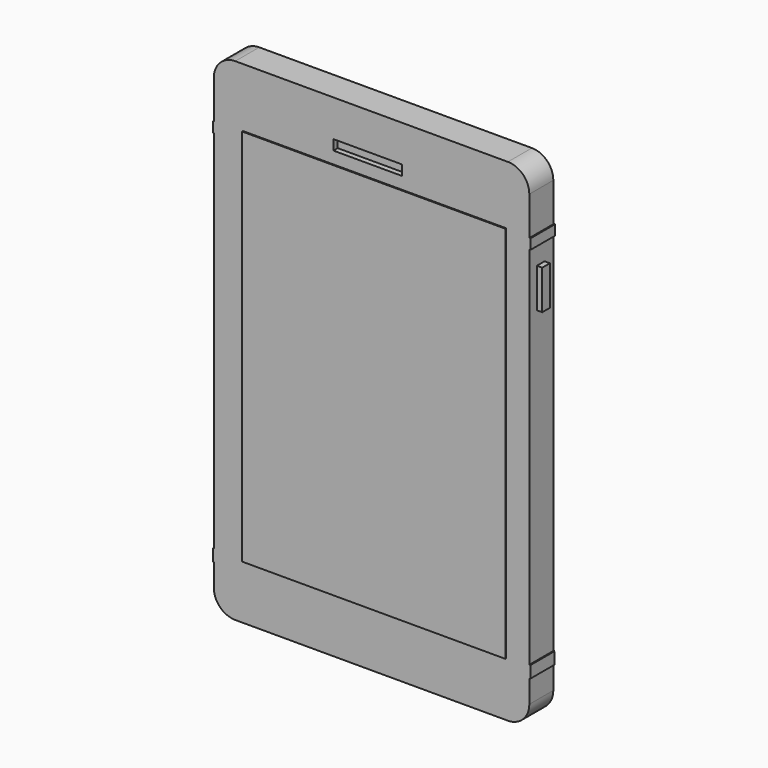
from build123d import *

# Parameters (mm, degrees)
F0_W      = 74.7929699719
F0_H      = 116.6311837733
F1_DEPTH  = 7.112
F2_W      = 2.2798741702
F2_H      = 9.3019269407
F3_DEPTH  = 1.27
F4_W      = 1.6649477184
F4_H      = 7.7697578818
F5_DEPTH  = 1.27
F4_H_2    = 7.214775309
F6_DEPTH  = 1.27
F4_W_2    = 1.2949595693
F4_H_3    = 4.4398605824
F7_DEPTH  = 0.508
F10_W     = 16.2794925272
F10_H     = 2.4049207568
F11_DEPTH = 1.27
F14_R     = 5.08
F15_R     = 5.08
F16_W     = 62.410261482
F16_H     = 89.7654034197
F17_DEPTH = 0.254
F21_R     = 5.3775746227
F22_DEPTH = 0.254
F25_W     = 74.7929699719
F25_H     = 2.4049244821
F26_DEPTH = 0.254
F29_DEPTH = 0.254
F30_DEPTH = 0.254
F31_W     = 74.7929699719
F31_H     = 2.9377117753
F34_DEPTH = 0.254
F32_W     = 7.112
F32_H     = 2.813577652
F35_DEPTH = 0.254
F33_W     = 7.112
F33_H     = 2.8514191508
F36_DEPTH = 0.254
F8_R      = 0.7916480681
F39_DEPTH = 1.27
F9_R      = 0.7862255443
F9_R_2    = 0.7916480681
F9_R_3    = 0.7862255169
F9_R_4    = 0.7902964021
F40_DEPTH = 1.27
F41_W     = 7.3253975715
F41_H     = 1.6351337545
F42_DEPTH = 1.27


# Not quite as in the source:
# - the program builds the solid bodies; features that only make, move or delete a surface that nothing else refers to are left out


with BuildPart() as f1:
    # F0 (on Front) → F1 (new body)
    with BuildSketch(Plane.XZ):
        with Locations((0.7164049894, -7.1640815586)):
            Rectangle(F0_W, F0_H)
    extrude(amount=F1_DEPTH)

    # F2 (on face) → F3 (join)
    with BuildSketch(Plane.YZ.offset(38.1128899753)):
        with Locations((-3.7364399759, 25.567272678)):
            Rectangle(F2_W, F2_H)
    extrude(amount=F3_DEPTH)

    # F4 (on face) → F5 (join)
    with BuildSketch(Plane(origin=(-36.6800799966, 0, 0), x_dir=(0, -1, 0), z_dir=(-1, 0, 0))):
        with Locations((2.8674099594, 15.4470177367)):
            Rectangle(F4_W, F4_H)
    extrude(amount=F5_DEPTH)

    # F4 (on face) → F6 (join)
    with BuildSketch(Plane(origin=(-36.6800799966, 0, 0), x_dir=(0, -1, 0), z_dir=(-1, 0, 0))):
        with Locations((2.8674099594, 27.5641391054)):
            Rectangle(F4_W, F4_H_2)
    extrude(amount=F6_DEPTH)

    # F4 (on face) → F7 (join)
    with BuildSketch(Plane(origin=(-36.6800799966, 0, 0), x_dir=(0, -1, 0), z_dir=(-1, 0, 0))):
        with Locations((3.052404034, 38.941282779)):
            Rectangle(F4_W_2, F4_H_3)
    extrude(amount=F7_DEPTH)

    # F10 (on face) → F11 (cut)
    with BuildSketch(Plane.XZ.offset(7.112)):
        with Locations((-0.1849941909, 41.2537120283)):
            Rectangle(F10_W, F10_H)
    extrude(amount=-F11_DEPTH, mode=Mode.SUBTRACT)

    # F14
    f14_edges = [f1.edges().sort_by_distance(p)[0] for p in [
        (38.11289, -3.556, 51.15151),
    ]]
    fillet(f14_edges, radius=F14_R)

    # F15
    f15_edges = [f1.edges().sort_by_distance(p)[0] for p in [
        (-36.68008, -3.556, 51.15151),
        (-36.68008, -3.556, -65.479673),
        (38.11289, -3.556, -65.479673),
    ]]
    fillet(f15_edges, radius=F15_R)

    # F16 (on face) → F17 (join)
    with BuildSketch(Plane.XZ.offset(7.112)):
        with Locations((1.43471919, -7.7157635242)):
            Rectangle(F16_W, F16_H)
    extrude(amount=F17_DEPTH)

    # F21 (on Front) → F22 (join)
    with BuildSketch(Plane.XZ):
        with Locations((30.1540587097, 43.5661412776)):
            Circle(F21_R)
    extrude(amount=-F22_DEPTH)

    # F25 (on face) → F26 (join)
    with BuildSketch(Plane(origin=(0, 0, 0), x_dir=(-1, 0, 0), z_dir=(0, 1, 0))):
        with Locations((-0.7164049894, 35.7038844377)):
            Rectangle(F25_W, F25_H)
    extrude(amount=F26_DEPTH)

    # F27 (on face) → F29 (join)
    with BuildSketch(Plane.YZ.offset(38.1128899753)):
        Polygon((0.254, 34.5014221966), (0.254, 36.9063466787), (0, 36.9063466787), (-7.112, 36.9063466787), (-7.112, 34.5014221966), (0, 34.5014221966), align=None)
    extrude(amount=F29_DEPTH)

    # F28 (on face) → F30 (join)
    with BuildSketch(Plane(origin=(-36.6800799966, 0, 0), x_dir=(0, -1, 0), z_dir=(-1, 0, 0))):
        Polygon((2.4049242493, 36.9063466787), (0, 36.9063466787), (-0.254, 36.9063466787), (-0.254, 34.5014221966), (0, 34.5014221966), (7.112, 34.5014221966), (7.112, 36.9063466787), (3.6998838186, 36.9063466787), (3.6998838186, 36.7213524878), (2.4049242493, 36.7213524878), align=None)
    extrude(amount=F30_DEPTH)

    # F31 (on face) → F34 (join)
    with BuildSketch(Plane(origin=(0, 0, 0), x_dir=(-1, 0, 0), z_dir=(0, 1, 0))):
        with Locations((-0.7164049894, -53.544729948)):
            Rectangle(F31_W, F31_H)
    extrude(amount=F34_DEPTH)

    # F32 (on face) → F35 (join)
    with BuildSketch(Plane.YZ.offset(38.1128899753)):
        with Locations((-3.556, -53.5610467196)):
            Rectangle(F32_W, F32_H)
    extrude(amount=F35_DEPTH)

    # F33 (on face) → F36 (join)
    with BuildSketch(Plane(origin=(-36.6800799966, 0, 0), x_dir=(0, -1, 0), z_dir=(-1, 0, 0))):
        with Locations((3.556, -53.6269359291)):
            Rectangle(F33_W, F33_H)
    extrude(amount=F36_DEPTH)

    # F8 (on face) → F39 (cut)
    with BuildSketch(Plane(origin=(0, 0, -65.4796734452), x_dir=(1, 0, 0), z_dir=(0, 0, -1))):
        with Locations((20.1854705811, 3.3230686095)):
            Circle(F8_R)
    extrude(amount=-F39_DEPTH, mode=Mode.SUBTRACT)

    # F9 (on face) → F40 (cut)
    with BuildSketch(Plane(origin=(0, 0, -65.4796734452), x_dir=(1, 0, 0), z_dir=(0, 0, -1))):
        with Locations((30.3601529449, 3.3230686095)):
            Circle(F9_R)
        with Locations((28.4177139401, 3.3230686095)):
            Circle(F9_R_2)
        with Locations((26.3827759773, 3.3230686095)):
            Circle(F9_R)
        with Locations((24.4403369725, 3.3230686095)):
            Circle(F9_R_3)
        with Locations((22.3591532558, 3.3230686095)):
            Circle(F9_R_4)
    extrude(amount=-F40_DEPTH, mode=Mode.SUBTRACT)

    # F41 (on face) → F42 (cut)
    with BuildSketch(Plane(origin=(0, 0, -65.4796734452), x_dir=(1, 0, 0), z_dir=(0, 0, -1))):
        with Locations((0.251334277, 2.8914771974)):
            Rectangle(F41_W, F41_H)
    extrude(amount=-F42_DEPTH, mode=Mode.SUBTRACT)


solid = f1.part
